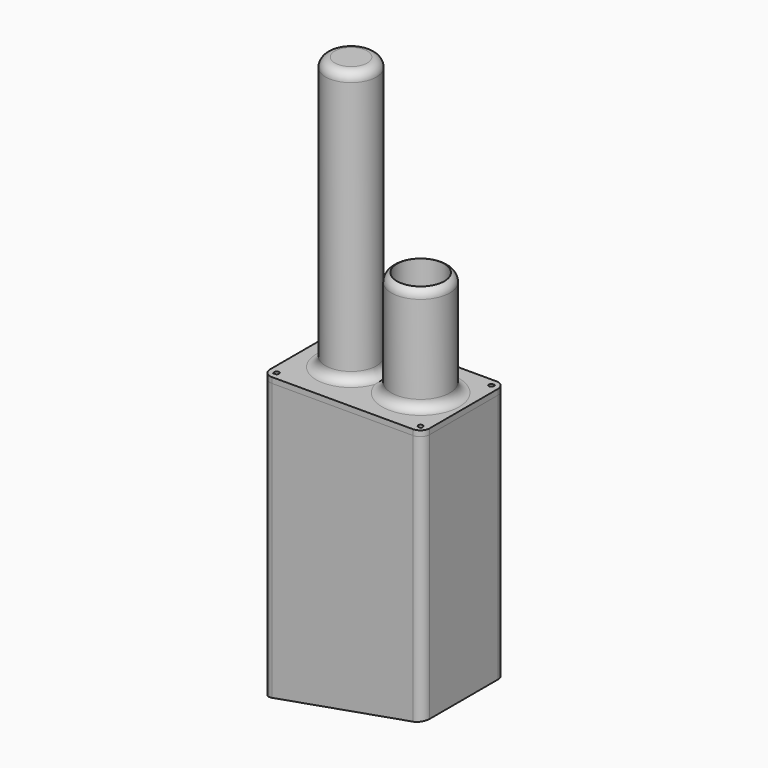
from build123d import *

# Parameters (mm, degrees)
F0_W         = 86
F0_H         = 56
F1_DEPTH     = 150
F2_DEPTH     = 30
F0_R         = 13.75
F0_R_2       = 15.75
F3_DEPTH     = 3
F0_R_3       = 12.75
F4_DEPTH     = 60
F5_DEPTH     = 150
F7_DEPTH     = 56.001
F8_R         = 5
F9_T9_DEPTH  = 28
F9_T11_DEPTH = 28
F9_T13_DEPTH = 28
F9_T15_DEPTH = 28


# Not quite as in the source:
# - a fillet or chamfer that OpenCascade refuses, or shapes differently, is made with other operations: its cross-section is extruded or revolved along the edge and cut away or added


with BuildPart() as f1:
    # F0 (on Top) → F1 (new body)
    with BuildSketch(Plane.XY):
        Rectangle(F0_W, F0_H)
        Polygon((-38.75, 25), (-34.6879807977, 25), (34.6879807977, 25), (38.75, 25), (40, 25), (40, 23.75), (40, 19.6879807977), (40, -19.6879807977), (40, -23.75), (40, -25), (38.75, -25), (34.6879807977, -25), (-34.6879807977, -25), (-38.75, -25), (-40, -25), (-40, -23.75), (-40, -19.6879807977), (-40, 19.6879807977), (-40, 23.75), (-40, 25), align=None, mode=Mode.SUBTRACT)
    extrude(amount=-F1_DEPTH)

    # F0 (on Top) → F2 (join)
    with BuildSketch(Plane.XY):
        with BuildLine():
            ThreePointArc((-40, 19.6879807977), (-35.74479618, 20.74479618), (-34.6879807977, 25))
            Line((-34.6879807977, 25), (-38.75, 25))
            ThreePointArc((-38.75, 25), (-37.8661165235, 24.6338834765), (-37.5, 23.75))
            ThreePointArc((-37.5, 23.75), (-38.75, 22.5), (-40, 23.75))
            Line((-40, 23.75), (-40, 19.6879807977))
        make_face()
        with BuildLine():
            Line((38.75, 25), (34.6879807977, 25))
            ThreePointArc((34.6879807977, 25), (35.74479618, 20.74479618), (40, 19.6879807977))
            Line((40, 19.6879807977), (40, 23.75))
            ThreePointArc((40, 23.75), (37.8661165235, 22.8661165235), (38.75, 25))
        make_face()
        with BuildLine():
            ThreePointArc((-34.6879807977, -25), (-35.74479618, -20.74479618), (-40, -19.6879807977))
            Line((-40, -19.6879807977), (-40, -23.75))
            ThreePointArc((-40, -23.75), (-38.75, -22.5), (-37.5, -23.75))
            ThreePointArc((-37.5, -23.75), (-37.8661165235, -24.6338834765), (-38.75, -25))
            Line((-38.75, -25), (-34.6879807977, -25))
        make_face()
        with BuildLine():
            Line((40, -23.75), (40, -19.6879807977))
            ThreePointArc((40, -19.6879807977), (35.74479618, -20.74479618), (34.6879807977, -25))
            Line((34.6879807977, -25), (38.75, -25))
            ThreePointArc((38.75, -25), (37.8661165235, -22.8661165235), (40, -23.75))
        make_face()
        with BuildLine():
            ThreePointArc((-40, 23.75), (-39.6338834765, 24.6338834765), (-38.75, 25))
            Line((-38.75, 25), (-40, 25))
            Line((-40, 25), (-40, 23.75))
        make_face()
        with BuildLine():
            Line((40, 25), (38.75, 25))
            ThreePointArc((38.75, 25), (39.6338834765, 24.6338834765), (40, 23.75))
            Line((40, 23.75), (40, 25))
        make_face()
        with BuildLine():
            Line((40, -25), (40, -23.75))
            ThreePointArc((40, -23.75), (39.6338834765, -24.6338834765), (38.75, -25))
            Line((38.75, -25), (40, -25))
        make_face()
        with BuildLine():
            ThreePointArc((-38.75, -25), (-39.6338834765, -24.6338834765), (-40, -23.75))
            Line((-40, -23.75), (-40, -25))
            Line((-40, -25), (-38.75, -25))
        make_face()
    extrude(amount=-F2_DEPTH)

    # F6 (on face) → F7 (cut, through all)
    with BuildSketch(Plane.XZ.offset(28)):
        Polygon((43, -134.8358796591), (-43, -150), (43, -150), align=None)
    extrude(amount=-F7_DEPTH, mode=Mode.SUBTRACT)

    # F8
    f8_edges = [f1.edges().sort_by_distance(p)[0] for p in [
        (-43, -28, -75),
        (43, -28, -67.41794),
        (-43, 28, -75),
        (43, 28, -67.41794),
    ]]
    fillet(f8_edges, radius=F8_R)


with BuildPart() as f3:
    # F0 (on Top) → F3 (new body)
    with BuildSketch(Plane.XY):
        Rectangle(F0_W, F0_H)
        Polygon((-38.75, 25), (-34.6879807977, 25), (34.6879807977, 25), (38.75, 25), (40, 25), (40, 23.75), (40, 19.6879807977), (40, -19.6879807977), (40, -23.75), (40, -25), (38.75, -25), (34.6879807977, -25), (-34.6879807977, -25), (-38.75, -25), (-40, -25), (-40, -23.75), (-40, -19.6879807977), (-40, 19.6879807977), (-40, 23.75), (-40, 25), align=None, mode=Mode.SUBTRACT)
        with BuildLine():
            Line((34.6879807977, 25), (-34.6879807977, 25))
            ThreePointArc((-34.6879807977, 25), (-35.74479618, 20.74479618), (-40, 19.6879807977))
            Line((-40, 19.6879807977), (-40, -19.6879807977))
            ThreePointArc((-40, -19.6879807977), (-35.74479618, -20.74479618), (-34.6879807977, -25))
            Line((-34.6879807977, -25), (34.6879807977, -25))
            ThreePointArc((34.6879807977, -25), (35.74479618, -20.74479618), (40, -19.6879807977))
            Line((40, -19.6879807977), (40, 19.6879807977))
            ThreePointArc((40, 19.6879807977), (35.74479618, 20.74479618), (34.6879807977, 25))
        make_face()
        with Locations((-17.75, 0)):
            Circle(F0_R, mode=Mode.SUBTRACT)
        with Locations((19.75, 0)):
            Circle(F0_R_2, mode=Mode.SUBTRACT)
        with BuildLine():
            ThreePointArc((-40, 19.6879807977), (-35.74479618, 20.74479618), (-34.6879807977, 25))
            Line((-34.6879807977, 25), (-38.75, 25))
            ThreePointArc((-38.75, 25), (-37.8661165235, 24.6338834765), (-37.5, 23.75))
            ThreePointArc((-37.5, 23.75), (-38.75, 22.5), (-40, 23.75))
            Line((-40, 23.75), (-40, 19.6879807977))
        make_face()
        with BuildLine():
            ThreePointArc((-34.6879807977, -25), (-35.74479618, -20.74479618), (-40, -19.6879807977))
            Line((-40, -19.6879807977), (-40, -23.75))
            ThreePointArc((-40, -23.75), (-38.75, -22.5), (-37.5, -23.75))
            ThreePointArc((-37.5, -23.75), (-37.8661165235, -24.6338834765), (-38.75, -25))
            Line((-38.75, -25), (-34.6879807977, -25))
        make_face()
        with BuildLine():
            Line((40, -23.75), (40, -19.6879807977))
            ThreePointArc((40, -19.6879807977), (35.74479618, -20.74479618), (34.6879807977, -25))
            Line((34.6879807977, -25), (38.75, -25))
            ThreePointArc((38.75, -25), (37.8661165235, -22.8661165235), (40, -23.75))
        make_face()
        with BuildLine():
            Line((38.75, 25), (34.6879807977, 25))
            ThreePointArc((34.6879807977, 25), (35.74479618, 20.74479618), (40, 19.6879807977))
            Line((40, 19.6879807977), (40, 23.75))
            ThreePointArc((40, 23.75), (37.8661165235, 22.8661165235), (38.75, 25))
        make_face()
    extrude(amount=F3_DEPTH)

    # F0 (on Top) → F4 (join)
    with BuildSketch(Plane.XY):
        with Locations((19.75, 0)):
            Circle(F0_R_2)
        with Locations((19.75, 0)):
            Circle(F0_R_3, mode=Mode.SUBTRACT)
    extrude(amount=F4_DEPTH)

    # F0 (on Top) → F5 (join)
    with BuildSketch(Plane.XY):
        with Locations((-17.75, 0)):
            Circle(F0_R)
    extrude(amount=F5_DEPTH)

    # F9: fillet of radius 5 on 8 edges, made by hand

    # F9_s1 → F9_t2 (revolve, cut)
    with BuildSketch(Plane.XZ):
        with BuildLine():
            ThreePointArc((35.5, 55.417424305), (34.6833001327, 58.1560370926), (32.5, 60))
            Line((32.5, 60), (35.5, 60))
            Line((35.5, 60), (35.5, 55.417424305))
        make_face()
    revolve(axis=Axis((19.75, 0, 60), (0, 0, 1)), mode=Mode.SUBTRACT)

    # F9_s3 → F9_t4 (revolve, cut)
    with BuildSketch(Plane.XZ):
        with BuildLine():
            ThreePointArc((-4, 145), (-5.4644660941, 148.5355339059), (-9, 150))
            Line((-9, 150), (-4, 150))
            Line((-4, 150), (-4, 145))
        make_face()
    revolve(axis=Axis((-17.75, 0, 150), (0, 0, 1)), mode=Mode.SUBTRACT)

    # F9_s5 → F9_t6 (revolve)
    with BuildSketch(Plane.XZ):
        with BuildLine():
            ThreePointArc((40.5, 3), (36.9644660941, 4.4644660941), (35.5, 8))
            Line((35.5, 8), (35.5, 3))
            Line((35.5, 3), (40.5, 3))
        make_face()
    revolve(axis=Axis((19.75, 0, 3), (0, 0, 1)))

    # F9_s7 → F9_t8 (revolve)
    with BuildSketch(Plane.XZ):
        with BuildLine():
            ThreePointArc((1, 3), (-2.5355339059, 4.4644660941), (-4, 8))
            Line((-4, 8), (-4, 3))
            Line((-4, 3), (1, 3))
        make_face()
    revolve(axis=Axis((-17.75, 0, 3), (0, 0, 1)))

    # F9_s10 → F9_t9 (cut)
    with BuildSketch(Plane.XY.offset(-12.5)):
        with BuildLine():
            ThreePointArc((-43, -23), (-41.5355339059, -26.5355339059), (-38, -28))
            Line((-38, -28), (-43, -28))
            Line((-43, -28), (-43, -23))
        make_face()
    extrude(amount=F9_T9_DEPTH, mode=Mode.SUBTRACT)

    # F9_s12 → F9_t11 (cut)
    with BuildSketch(Plane.XY.offset(-12.5)):
        with BuildLine():
            ThreePointArc((43, -23), (41.5355339059, -26.5355339059), (38, -28))
            Line((38, -28), (43, -28))
            Line((43, -28), (43, -23))
        make_face()
    extrude(amount=F9_T11_DEPTH, mode=Mode.SUBTRACT)

    # F9_s14 → F9_t13 (cut)
    with BuildSketch(Plane.XY.offset(-12.5)):
        with BuildLine():
            ThreePointArc((-38, 28), (-41.5355339059, 26.5355339059), (-43, 23))
            Line((-43, 23), (-43, 28))
            Line((-43, 28), (-38, 28))
        make_face()
    extrude(amount=F9_T13_DEPTH, mode=Mode.SUBTRACT)

    # F9_s16 → F9_t15 (cut)
    with BuildSketch(Plane.XY.offset(-12.5)):
        with BuildLine():
            ThreePointArc((38, 28), (41.5355339059, 26.5355339059), (43, 23))
            Line((43, 23), (43, 28))
            Line((43, 28), (38, 28))
        make_face()
    extrude(amount=F9_T15_DEPTH, mode=Mode.SUBTRACT)


solid = Compound([f1.part, f3.part])
